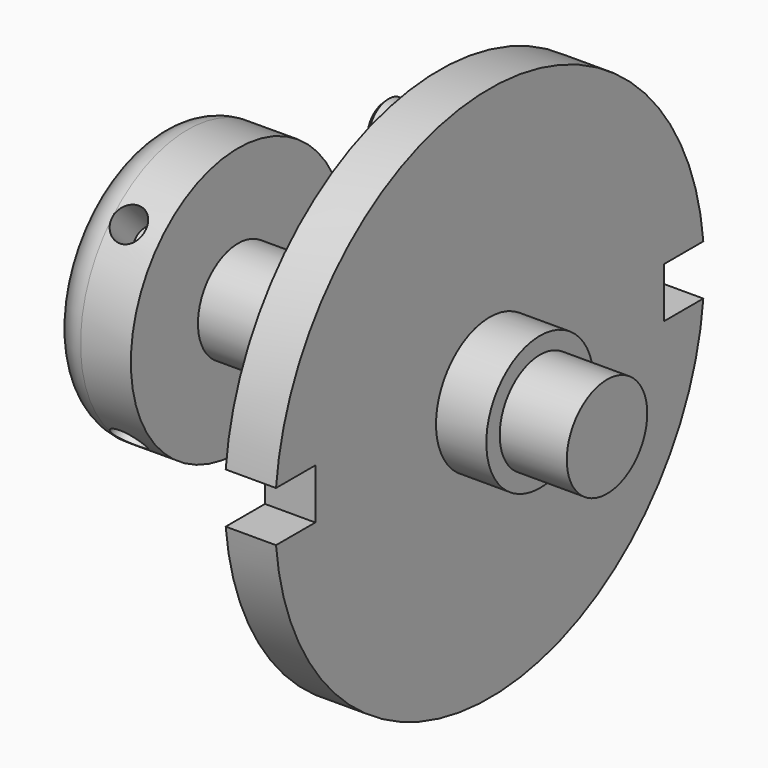
from build123d import *

# Parameters (mm, degrees)
F3_DEPTH        = 25.4
F4_R            = 9.525
F5_DEPTH        = 20.828
F6_SIZE         = 1.5875
F9_COPIES_COUNT = 4


# Not quite as in the source:
# - a pattern or mirror of a feature is missing from the dataset's text; its kind, count and spacing are read off the source's solid


with BuildPart() as f1:
    # F0 (on Top) → F1 (revolve)
    with BuildSketch(Plane.XY):
        with BuildLine():
            Line((-85.725, 38.1), (-85.725, 0))
            Line((-85.725, 0), (85.725, 0))
            Line((85.725, 0), (85.725, 19.05))
            Line((85.725, 19.05), (60.325, 19.05))
            Line((60.325, 19.05), (60.325, 25.4))
            Line((60.325, 25.4), (41.275, 25.4))
            Line((41.275, 25.4), (41.275, 101.6))
            Line((41.275, 101.6), (22.225, 101.6))
            Line((22.225, 101.6), (22.225, 19.05))
            Line((22.225, 19.05), (-53.975, 19.05))
            Line((-53.975, 19.05), (-53.975, 50.8))
            Line((-53.975, 50.8), (-73.025, 50.8))
            ThreePointArc((-73.025, 50.8), (-82.0052561211, 47.0802561211), (-85.725, 38.1))
        make_face()
    revolve(axis=Axis((0, 0, 0), (1, 0, 0)))

    # F2 (on face) → F3 (cut)
    with BuildSketch(Plane(origin=(22.225, 0, 0), x_dir=(0, -1, 0), z_dir=(-1, 0, 0))):
        with BuildLine():
            ThreePointArc((-101.1525302452, -9.525), (-101.6, 0), (-101.1525302452, 9.525))
            Line((-101.1525302452, 9.525), (-107.95, 9.525))
            Line((-107.95, 9.525), (-107.95, -9.525))
            Line((-107.95, -9.525), (-101.1525302452, -9.525))
        make_face()
        with BuildLine():
            ThreePointArc((101.1525302452, 9.525), (101.4880709071, 4.7677524627), (101.6, 0))
            ThreePointArc((101.6, 0), (101.4880709071, -4.7677524627), (101.1525302452, -9.525))
            Line((101.1525302452, -9.525), (107.95, -9.525))
            Line((107.95, -9.525), (107.95, 9.525))
            Line((107.95, 9.525), (101.1525302452, 9.525))
        make_face()
        with BuildLine():
            ThreePointArc((101.1525302452, -9.525), (101.4880709071, -4.7677524627), (101.6, 0))
            ThreePointArc((101.6, 0), (101.4880709071, 4.7677524627), (101.1525302452, 9.525))
            Line((101.1525302452, 9.525), (82.55, 9.525))
            Line((82.55, 9.525), (82.55, -9.525))
            Line((82.55, -9.525), (101.1525302452, -9.525))
        make_face()
        with BuildLine():
            Line((-82.55, 9.525), (-101.1525302452, 9.525))
            ThreePointArc((-101.1525302452, 9.525), (-101.6, 0), (-101.1525302452, -9.525))
            Line((-101.1525302452, -9.525), (-82.55, -9.525))
            Line((-82.55, -9.525), (-82.55, 9.525))
        make_face()
    extrude(amount=-F3_DEPTH, mode=Mode.SUBTRACT)

    # F4 (on face) → F5 (join)
    with BuildSketch(Plane(origin=(22.225, 0, 0), x_dir=(0, -1, 0), z_dir=(-1, 0, 0))):
        with Locations((0, 76.2)):
            Circle(F4_R)
        with Locations((0, -76.2)):
            Circle(F4_R)
    extrude(amount=F5_DEPTH)

    # F6
    f6_edges = [f1.edges().sort_by_distance(p)[0] for p in [
        (1.397, 9.525, 76.2),
        (1.397, 9.525, -76.2),
    ]]
    chamfer(f6_edges, length=F6_SIZE)

    # F8 (on offset) → F9 (revolve, cut)
    with BuildSketch(Plane.YZ.offset(-66.675)):
        Polygon((24.6957043329, -24.6957043329), (35.9210244843, -35.9210244843), (39.5131269327, -39.5131269327), (44.0032549932, -35.0229988722), (29.1858323935, -20.2055762724), align=None)
    f9 = revolve(axis=Axis((-66.675, 30.3083644086, -30.3083644086), (0, -0.7071067812, 0.7071067812)), mode=Mode.SUBTRACT)

    # F9_copies: F9 ×4 about axis
    f9_copies_axis = Axis((0, 0, 0), (1, 0, 0))
    for i in range(1, F9_COPIES_COUNT):
        add(f9.rotate(f9_copies_axis, i * 360 / F9_COPIES_COUNT), mode=Mode.SUBTRACT)


solid = f1.part
